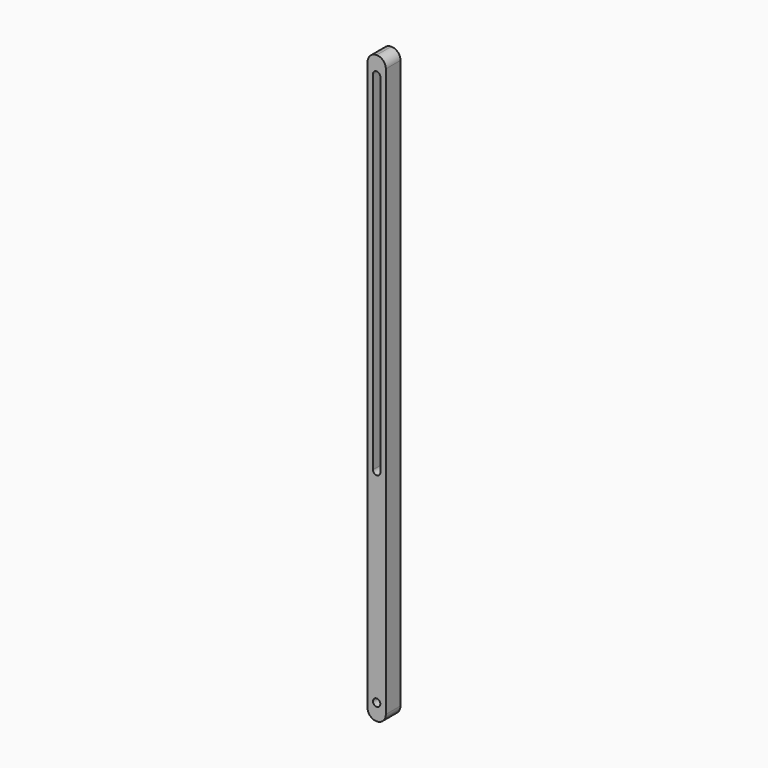
from build123d import *

# Parameters (mm, degrees)
F0_W     = 25
F0_H     = 800
F1_DEPTH = 25
F2_W     = 10
F2_H     = 475
F3_DEPTH = 25
F4_R     = 5
F5_DEPTH = 25
F7_DEPTH = 25
F9_DEPTH = 25
F10_R    = 12.49999
F11_R    = 12.49999


# Not quite as in the source:
# - a fillet or chamfer is up to 0.001 mm smaller than in the source, because OpenCascade refuses the exact size


with BuildPart() as f1:
    # F0 (on Front) → F1 (new body)
    with BuildSketch(Plane.XZ):
        Rectangle(F0_W, F0_H)
    extrude(amount=F1_DEPTH)

    # F2 (on face) → F3 (cut)
    with BuildSketch(Plane.XZ.offset(25)):
        with Locations((0, 138.0000114441)):
            Rectangle(F2_W, F2_H)
    extrude(amount=-F3_DEPTH, mode=Mode.SUBTRACT)

    # F4 (on face) → F5 (cut)
    with BuildSketch(Plane.XZ.offset(25)):
        with Locations((0, -377.3987293243)):
            Circle(F4_R)
    extrude(amount=-F5_DEPTH, mode=Mode.SUBTRACT)

    # F6 (on face) → F7 (cut)
    with BuildSketch(Plane.XZ.offset(25)):
        with BuildLine():
            Line((-5, 375.5000114441), (5, 375.5000114441))
            ThreePointArc((5, 375.5000114441), (0, 380.5000114441), (-5, 375.5000114441))
        make_face()
    extrude(amount=-F7_DEPTH, mode=Mode.SUBTRACT)

    # F8 (on face) → F9 (cut)
    with BuildSketch(Plane.XZ.offset(25)):
        with BuildLine():
            Line((5, -99.4999885559), (-5, -99.4999885559))
            ThreePointArc((-5, -99.4999885559), (0, -104.4999885559), (5, -99.4999885559))
        make_face()
    extrude(amount=-F9_DEPTH, mode=Mode.SUBTRACT)

    # F10 (radius 12.5 in the source; OpenCascade refuses exactly that, so slightly less here)
    f10_edges = [f1.edges().sort_by_distance(p)[0] for p in [
        (-12.5, -12.5, 400),
        (12.5, -12.5, 400),
    ]]
    fillet(f10_edges, radius=F10_R)

    # F11 (radius 12.5 in the source; OpenCascade refuses exactly that, so slightly less here)
    f11_edges = [f1.edges().sort_by_distance(p)[0] for p in [
        (-12.5, -12.5, -400),
        (12.5, -12.5, -400),
    ]]
    fillet(f11_edges, radius=F11_R)


solid = f1.part
